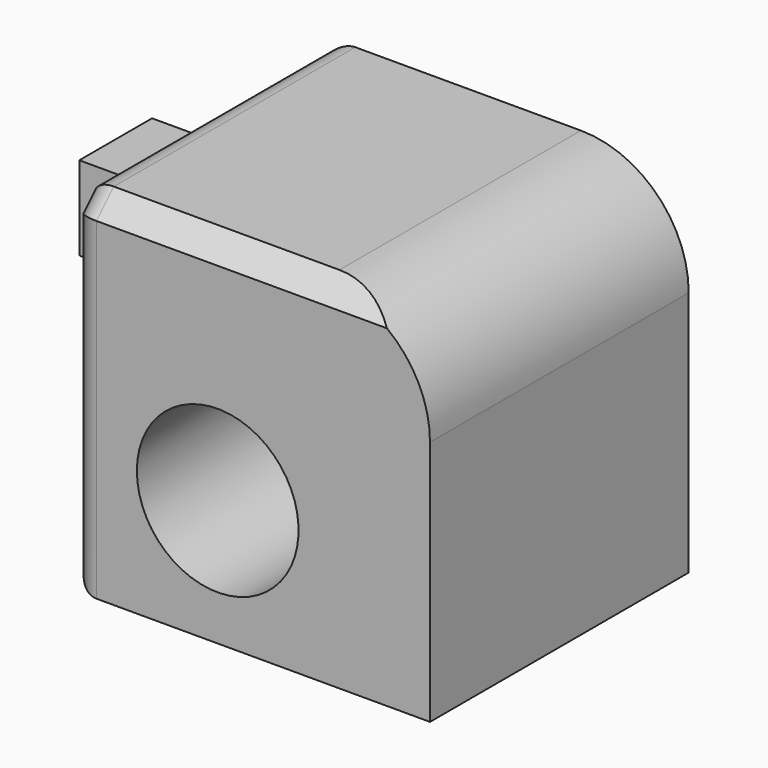
from build123d import *

# Parameters (mm, degrees)
F0_W          = 84.9268175662
F0_H          = 83.4368709475
F1_DEPTH      = 76.2
F2_SIZE       = 5.08
F3_R          = 25.4
F5_D          = 38.1
F8_T          = -2.54
F9_W          = 21.4254707098
F9_H          = 19.7638887912
F10_DEPTH     = 25.4
F11_T1_DEPTH  = 19.7638887912
F11_T3_DEPTH  = 21.4254707098
F11_T9_DEPTH  = 35.6388887912
F11_T13_DEPTH = 37.3004707098
F11_T20_DEPTH = 35.6388887912
F11_T24_DEPTH = 37.3004707098
F11_T31_DEPTH = 37.3004707098
F11_T35_DEPTH = 35.6388887912
F11_T42_DEPTH = 35.6388887912
F11_T46_DEPTH = 37.3004707098
F11_T49_DEPTH = 102.87
F11_T51_DEPTH = 38.9342048969
F11_T53_DEPTH = 115.1868709475
F11_T55_DEPTH = 110.1068709475
F11_T57_DEPTH = 107.95


# Not quite as in the source:
# - a fillet or chamfer that OpenCascade refuses, or shapes differently, is made with other operations: its cross-section is extruded or revolved along the edge and cut away or added


with BuildPart() as f1:
    # F0 (on Front) → F1 (new body)
    with BuildSketch(Plane.XZ):
        with Locations((-3.4268703312, 12.0685463771)):
            Rectangle(F0_W, F0_H)
    extrude(amount=F1_DEPTH)

    # F2
    f2_edges = [f1.edges().sort_by_distance(p)[0] for p in [
        (-3.42687, -76.2, 53.786982),
    ]]
    chamfer(f2_edges, length=F2_SIZE)

    # F3
    f3_edges = [f1.edges().sort_by_distance(p)[0] for p in [
        (39.036538, -35.56, 53.786982),
    ]]
    fillet(f3_edges, radius=F3_R)

    # F5 (through all)
    with Locations(Plane.XZ.offset(76.2)):
        with Locations((-10.9889917076, 0)):
            Hole(F5_D / 2)

    # F8
    f8_openings = [f1.faces().sort_by_distance(p)[0] for p in [
        (-16.12687, 0, 52.596424),
    ]]
    offset(amount=F8_T, openings=f8_openings)

    # F9 (on face) → F10 (join)
    with BuildSketch(Plane(origin=(-45.8902791142, 0, 0), x_dir=(0, -1, 0), z_dir=(-1, 0, 0))):
        with Locations((30.8794565499, 27.0300125703)):
            Rectangle(F9_W, F9_H)
    extrude(amount=F10_DEPTH)

    # F11: fillet of radius 6.35 on 9 edges, made by hand

    # F11_s2 → F11_t1 (join)
    with BuildSketch(Plane.XY.offset(17.1480681747)):
        with BuildLine():
            ThreePointArc((-45.8902791142, -13.816721195), (-47.7501510537, -18.3068492555), (-52.2402791142, -20.166721195))
            Line((-52.2402791142, -20.166721195), (-45.8902791142, -20.166721195))
            Line((-45.8902791142, -20.166721195), (-45.8902791142, -13.816721195))
        make_face()
        with BuildLine():
            ThreePointArc((-45.8902791142, -47.9421919048), (-47.7501510537, -43.4520638442), (-52.2402791142, -41.5921919048))
            Line((-52.2402791142, -41.5921919048), (-45.8902791142, -41.5921919048))
            Line((-45.8902791142, -41.5921919048), (-45.8902791142, -47.9421919048))
        make_face()
    extrude(amount=F11_T1_DEPTH)

    # F11_s4 → F11_t3 (join)
    with BuildSketch(Plane.XZ.offset(20.166721195)):
        with BuildLine():
            ThreePointArc((-45.8902791142, 43.2619569659), (-47.7501510537, 38.7718289054), (-52.2402791142, 36.9119569659))
            Line((-52.2402791142, 36.9119569659), (-45.8902791142, 36.9119569659))
            Line((-45.8902791142, 36.9119569659), (-45.8902791142, 43.2619569659))
        make_face()
        with BuildLine():
            ThreePointArc((-45.8902791142, 10.7980681747), (-47.7501510537, 15.2881962353), (-52.2402791142, 17.1480681747))
            Line((-52.2402791142, 17.1480681747), (-45.8902791142, 17.1480681747))
            Line((-45.8902791142, 17.1480681747), (-45.8902791142, 10.7980681747))
        make_face()
    extrude(amount=F11_T3_DEPTH)


with BuildPart() as f11_tool7:
    # F11_s8 → F11_t9 (new body)
    with BuildSketch(Plane.XY.offset(52.7869569659)):
        with BuildLine():
            ThreePointArc((-45.8902791142, -13.816721195), (-47.7501510537, -18.3068492555), (-52.2402791142, -20.166721195))
            Line((-52.2402791142, -20.166721195), (-45.8902791142, -20.166721195))
            Line((-45.8902791142, -20.166721195), (-45.8902791142, -13.816721195))
        make_face()
    extrude(amount=-F11_T9_DEPTH)

    split(bisect_by=Plane.XY.offset(36.9119569659), keep=Keep.TOP)


with BuildPart() as f11_tool11:
    # F11_s12 → F11_t13 (new body)
    with BuildSketch(Plane.XZ.offset(41.5921919048)):
        with BuildLine():
            ThreePointArc((-45.8902791142, 43.2619569659), (-47.7501510537, 38.7718289054), (-52.2402791142, 36.9119569659))
            Line((-52.2402791142, 36.9119569659), (-45.8902791142, 36.9119569659))
            Line((-45.8902791142, 36.9119569659), (-45.8902791142, 43.2619569659))
        make_face()
    extrude(amount=-F11_T13_DEPTH)

    split(bisect_by=Plane.XZ.offset(20.166721195), keep=Keep.BOTTOM)


with BuildPart() as f11_tool7_1:
    add(f11_tool7.part)

    # F11_t15: intersect F11_tool11
    add(f11_tool11.part, mode=Mode.INTERSECT)


with BuildPart() as f1_1:
    add(f1.part)

    # F11_t5: union F11_tool7
    add(f11_tool7_1.part)


with BuildPart() as f11_tool18:
    # F11_s19 → F11_t20 (new body)
    with BuildSketch(Plane.XY.offset(36.9119569659)):
        with BuildLine():
            ThreePointArc((-45.8902791142, -13.816721195), (-47.7501510537, -18.3068492555), (-52.2402791142, -20.166721195))
            Line((-52.2402791142, -20.166721195), (-45.8902791142, -20.166721195))
            Line((-45.8902791142, -20.166721195), (-45.8902791142, -13.816721195))
        make_face()
    extrude(amount=-F11_T20_DEPTH)

    split(bisect_by=Plane.XY.offset(17.1480681747), keep=Keep.BOTTOM)


with BuildPart() as f11_tool22:
    # F11_s23 → F11_t24 (new body)
    with BuildSketch(Plane.XZ.offset(4.291721195)):
        with BuildLine():
            ThreePointArc((-45.8902791142, 10.7980681747), (-47.7501510537, 15.2881962353), (-52.2402791142, 17.1480681747))
            Line((-52.2402791142, 17.1480681747), (-45.8902791142, 17.1480681747))
            Line((-45.8902791142, 17.1480681747), (-45.8902791142, 10.7980681747))
        make_face()
    extrude(amount=F11_T24_DEPTH)

    split(bisect_by=Plane.XZ.offset(20.166721195), keep=Keep.BOTTOM)


with BuildPart() as f11_tool18_1:
    add(f11_tool18.part)

    # F11_t26: intersect F11_tool22
    add(f11_tool22.part, mode=Mode.INTERSECT)


with BuildPart() as f1_2:
    add(f1_1.part)

    # F11_t16: union F11_tool18
    add(f11_tool18_1.part)


with BuildPart() as f11_tool29:
    # F11_s30 → F11_t31 (new body)
    with BuildSketch(Plane.XZ.offset(57.4671919048)):
        with BuildLine():
            ThreePointArc((-45.8902791142, 43.2619569659), (-47.7501510537, 38.7718289054), (-52.2402791142, 36.9119569659))
            Line((-52.2402791142, 36.9119569659), (-45.8902791142, 36.9119569659))
            Line((-45.8902791142, 36.9119569659), (-45.8902791142, 43.2619569659))
        make_face()
    extrude(amount=-F11_T31_DEPTH)

    split(bisect_by=Plane.XZ.offset(41.5921919048), keep=Keep.TOP)


with BuildPart() as f11_tool33:
    # F11_s34 → F11_t35 (new body)
    with BuildSketch(Plane.XY.offset(17.1480681747)):
        with BuildLine():
            ThreePointArc((-45.8902791142, -47.9421919048), (-47.7501510537, -43.4520638442), (-52.2402791142, -41.5921919048))
            Line((-52.2402791142, -41.5921919048), (-45.8902791142, -41.5921919048))
            Line((-45.8902791142, -41.5921919048), (-45.8902791142, -47.9421919048))
        make_face()
    extrude(amount=F11_T35_DEPTH)

    split(bisect_by=Plane.XY.offset(36.9119569659), keep=Keep.TOP)


with BuildPart() as f11_tool29_1:
    add(f11_tool29.part)

    # F11_t37: intersect F11_tool33
    add(f11_tool33.part, mode=Mode.INTERSECT)


with BuildPart() as f1_3:
    add(f1_2.part)

    # F11_t27: union F11_tool29
    add(f11_tool29_1.part)


with BuildPart() as f11_tool40:
    # F11_s41 → F11_t42 (new body)
    with BuildSketch(Plane.XY.offset(1.2730681747)):
        with BuildLine():
            ThreePointArc((-45.8902791142, -47.9421919048), (-47.7501510537, -43.4520638442), (-52.2402791142, -41.5921919048))
            Line((-52.2402791142, -41.5921919048), (-45.8902791142, -41.5921919048))
            Line((-45.8902791142, -41.5921919048), (-45.8902791142, -47.9421919048))
        make_face()
    extrude(amount=F11_T42_DEPTH)

    split(bisect_by=Plane.XY.offset(17.1480681747), keep=Keep.BOTTOM)


with BuildPart() as f11_tool44:
    # F11_s45 → F11_t46 (new body)
    with BuildSketch(Plane.XZ.offset(20.166721195)):
        with BuildLine():
            ThreePointArc((-45.8902791142, 10.7980681747), (-47.7501510537, 15.2881962353), (-52.2402791142, 17.1480681747))
            Line((-52.2402791142, 17.1480681747), (-45.8902791142, 17.1480681747))
            Line((-45.8902791142, 17.1480681747), (-45.8902791142, 10.7980681747))
        make_face()
    extrude(amount=F11_T46_DEPTH)

    split(bisect_by=Plane.XZ.offset(41.5921919048), keep=Keep.TOP)


with BuildPart() as f11_tool40_1:
    add(f11_tool40.part)

    # F11_t48: intersect F11_tool44
    add(f11_tool44.part, mode=Mode.INTERSECT)


with BuildPart() as f1_4:
    add(f1_3.part)

    # F11_t38: union F11_tool40
    add(f11_tool40_1.part)

    # F11_s50 → F11_t49 (cut)
    with BuildSketch(Plane.XZ.offset(-15.875)):
        with BuildLine():
            ThreePointArc((-39.5402791142, 53.7869818509), (-44.0304071748, 51.9271099114), (-45.8902791142, 47.4369818509))
            Line((-45.8902791142, 47.4369818509), (-45.8902791142, 53.7869818509))
            Line((-45.8902791142, 53.7869818509), (-39.5402791142, 53.7869818509))
        make_face()
    extrude(amount=F11_T49_DEPTH, mode=Mode.SUBTRACT)

    # F11_s52 → F11_t51 (cut)
    with BuildSketch(Plane(origin=(0, 2.5588110768, 2.5588110768), x_dir=(1, 0, 0), z_dir=(0, -0.7071067812, -0.7071067812))):
        with BuildLine():
            ThreePointArc((-45.8902791142, 81.9725738843), (-44.0304071748, 86.4627019448), (-39.5402791142, 88.3225738843))
            Line((-39.5402791142, 88.3225738843), (-45.8902791142, 88.3225738843))
            Line((-45.8902791142, 88.3225738843), (-45.8902791142, 81.9725738843))
        make_face()
    extrude(amount=F11_T51_DEPTH, mode=Mode.SUBTRACT)

    # F11_s54 → F11_t53 (cut)
    with BuildSketch(Plane.XY.offset(-45.5248890966)):
        with BuildLine():
            ThreePointArc((-39.5402791142, 0), (-44.0304071748, -1.8598719395), (-45.8902791142, -6.35))
            Line((-45.8902791142, -6.35), (-45.8902791142, 0))
            Line((-45.8902791142, 0), (-39.5402791142, 0))
        make_face()
    extrude(amount=F11_T53_DEPTH, mode=Mode.SUBTRACT)

    # F11_s56 → F11_t55 (cut)
    with BuildSketch(Plane.XY.offset(-45.5248890966)):
        with BuildLine():
            ThreePointArc((-39.5402791142, -76.2), (-44.0304071748, -74.3401280605), (-45.8902791142, -69.85))
            Line((-45.8902791142, -69.85), (-45.8902791142, -76.2))
            Line((-45.8902791142, -76.2), (-39.5402791142, -76.2))
        make_face()
    extrude(amount=F11_T55_DEPTH, mode=Mode.SUBTRACT)

    # F11_s58 → F11_t57 (cut)
    with BuildSketch(Plane.XZ.offset(-15.875)):
        with BuildLine():
            ThreePointArc((-39.5402791142, -29.6498890966), (-44.0304071748, -27.7900171572), (-45.8902791142, -23.2998890966))
            Line((-45.8902791142, -23.2998890966), (-45.8902791142, -29.6498890966))
            Line((-45.8902791142, -29.6498890966), (-39.5402791142, -29.6498890966))
        make_face()
    extrude(amount=F11_T57_DEPTH, mode=Mode.SUBTRACT)


solid = f1_4.part
